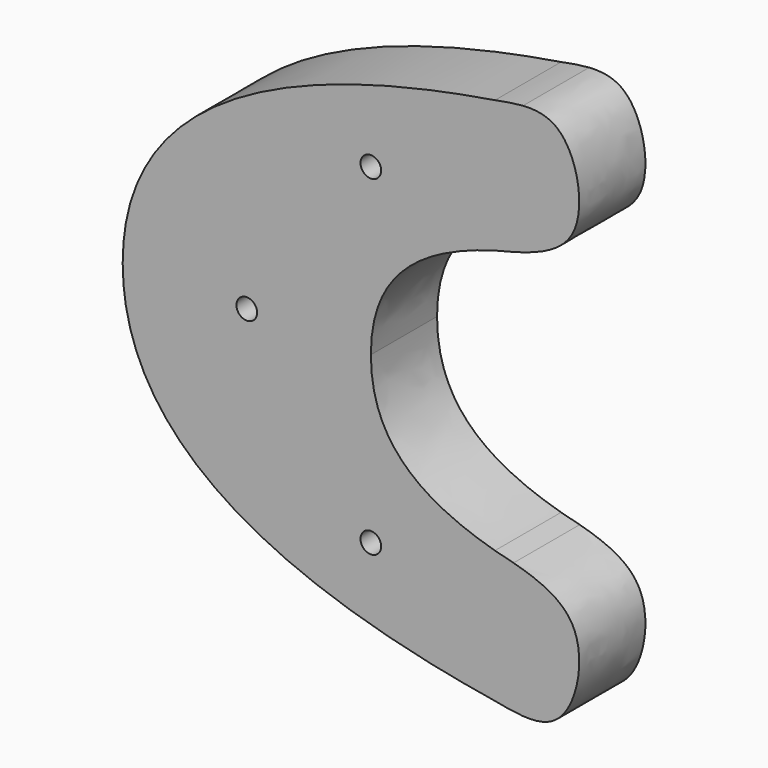
from build123d import *

# Parameters (mm, degrees)
F0_R     = 3.175
F1_DEPTH = 25.4


# Not quite as in the source:
# - ends of sketch curves that miss each other by under 0.0002 mm in the source are joined


with BuildPart() as f1:
    # F0 (on Front) → F1 (new body)
    with BuildSketch(Plane.XZ):
        with BuildLine():
            add(Edge.make_bspline(
                [(-228.6, 0), (-228.603328408, -20.9998549914), (-216.1362353399, -33.3187275092), (-190.5048638582, -40.5451878905)],
                knots=[0, 0, 0, 0, 96.8546122477, 96.8546122477, 96.8546122477, 96.8546122477], degree=3))
            add(Edge.make_bspline(
                [(-228.6, 0), (-228.603328408, 20.9998549914), (-216.1362353399, 33.3187275092), (-190.5048638582, 40.5451878905)],
                knots=[0, 0, 0, 0, 96.8546122477, 96.8546122477, 96.8546122477, 96.8546122477], degree=3))
            add(Edge.make_bspline(
                [(-190.5048638582, 40.5451878905), (-188.6690340196, 41.0627782819), (-186.7656708429, 41.5542443707), (-184.7945193799, 42.0209047272)],
                knots=[96.8546122477, 96.8546122477, 96.8546122477, 96.8546122477, 103.7917590678, 103.7917590678, 103.7917590678, 103.7917590678], degree=3))
            add(Edge.make_bspline(
                [(-181.8914412177, 82.4957251162), (-177.7740978469, 82.7671917451), (-166.6388871368, 81.1057466034), (-160.4841015231, 50.6684396177), (-176.6492852244, 44.2605429862), (-184.7945193799, 42.0209047272)],
                knots=[0.1201664208, 0.1201664208, 0.1201664208, 0.1201664208, 0.2987042421, 0.6454715168, 0.9336630859, 0.9336630859, 0.9336630859, 0.9336630859], degree=3))
            add(Edge.make_bspline(
                [(-190.5065755272, 81.190021553), (-187.6562706797, 81.6501805926), (-184.7832793111, 82.0849710788), (-181.8914412177, 82.4957251162)],
                knots=[152.2718692701, 152.2718692701, 152.2718692701, 152.2718692701, 159.2026765547, 159.2026765547, 159.2026765547, 159.2026765547], degree=3))
            add(Edge.make_bspline(
                [(-304.7999998765, 0.0020627141), (-304.7970834826, 48.7263819663), (-253.1268418931, 71.0804777771), (-190.5065755272, 81.190021553)],
                knots=[0.0042973705, 0.0042973705, 0.0042973705, 0.0042973705, 152.2718692701, 152.2718692701, 152.2718692701, 152.2718692701], degree=3))
            add(Edge.make_bspline(
                [(-304.8, -0.0020627142), (-304.8, -0.0006875504), (-304.7999999588, 0.0006875924), (-304.7999998765, 0.0020627141)],
                knots=[0, 0, 0, 0, 0.0042973705, 0.0042973705, 0.0042973705, 0.0042973705], degree=3))
            add(Edge.make_bspline(
                [(-304.8, -0.0020627142), (-304.7970834826, -48.7263819663), (-253.1268418931, -71.0804777771), (-190.5065755272, -81.190021553)],
                knots=[0.0042973705, 0.0042973705, 0.0042973705, 0.0042973705, 152.2718692701, 152.2718692701, 152.2718692701, 152.2718692701], degree=3))
            add(Edge.make_bspline(
                [(-190.5065755272, -81.190021553), (-187.6562706797, -81.6501805926), (-184.7832793111, -82.0849710788), (-181.8914412177, -82.4957251162)],
                knots=[152.2718692701, 152.2718692701, 152.2718692701, 152.2718692701, 159.2026765547, 159.2026765547, 159.2026765547, 159.2026765547], degree=3))
            add(Edge.make_bspline(
                [(-181.8914412177, -82.4957251162), (-177.7740978469, -82.7671917451), (-166.6388871368, -81.1057466034), (-160.4841015231, -50.6684396177), (-176.6492852244, -44.2605429862), (-184.7945193799, -42.0209047272)],
                knots=[0.1201664208, 0.1201664208, 0.1201664208, 0.1201664208, 0.2987042421, 0.6454715168, 0.9336630859, 0.9336630859, 0.9336630859, 0.9336630859], degree=3))
            add(Edge.make_bspline(
                [(-190.5048638582, -40.5451878905), (-188.6690340196, -41.0627782819), (-186.7656708429, -41.5542443707), (-184.7945193799, -42.0209047272)],
                knots=[96.8546122477, 96.8546122477, 96.8546122477, 96.8546122477, 103.7917590678, 103.7917590678, 103.7917590678, 103.7917590678], degree=3))
        make_face()
        with Locations((-228.6080516329, -50.8)):
            Circle(F0_R, mode=Mode.SUBTRACT)
        with Locations((-266.7, 0)):
            Circle(F0_R, mode=Mode.SUBTRACT)
        with Locations((-228.6080516329, 50.8)):
            Circle(F0_R, mode=Mode.SUBTRACT)
        with BuildLine():
            add(Edge.make_bspline(
                [(-190.5048638582, 40.5451878905), (-188.6690340196, 41.0627782819), (-186.7656708429, 41.5542443707), (-184.7945193799, 42.0209047272)],
                knots=[96.8546122477, 96.8546122477, 96.8546122477, 96.8546122477, 103.7917590678, 103.7917590678, 103.7917590678, 103.7917590678], degree=3))
            add(Edge.make_bspline(
                [(-184.7945193799, 42.0209047272), (-186.6694170397, 41.5053771867), (-188.587140449, 41.0252825386), (-190.5048638582, 40.5451878905)],
                knots=[0.9336630859, 0.9336630859, 0.9336630859, 0.9336630859, 1, 1, 1, 1], degree=3))
        make_face()
        with BuildLine():
            add(Edge.make_bspline(
                [(-184.7945193799, -42.0209047272), (-186.6694170397, -41.5053771867), (-188.587140449, -41.0252825386), (-190.5048638582, -40.5451878905)],
                knots=[0.9336630859, 0.9336630859, 0.9336630859, 0.9336630859, 1, 1, 1, 1], degree=3))
            add(Edge.make_bspline(
                [(-190.5048638582, -40.5451878905), (-188.6690340196, -41.0627782819), (-186.7656708429, -41.5542443707), (-184.7945193799, -42.0209047272)],
                knots=[96.8546122477, 96.8546122477, 96.8546122477, 96.8546122477, 103.7917590678, 103.7917590678, 103.7917590678, 103.7917590678], degree=3))
        make_face()
        with BuildLine():
            add(Edge.make_bspline(
                [(-190.5065755272, 81.190021553), (-187.6562706797, 81.6501805926), (-184.7832793111, 82.0849710788), (-181.8914412177, 82.4957251162)],
                knots=[152.2718692701, 152.2718692701, 152.2718692701, 152.2718692701, 159.2026765547, 159.2026765547, 159.2026765547, 159.2026765547], degree=3))
            add(Edge.make_bspline(
                [(-190.5065755272, 81.190021553), (-187.58461511, 81.7515168563), (-184.6626546928, 82.3130121597), (-181.8914412177, 82.4957251162)],
                knots=[0, 0, 0, 0, 0.1201664208, 0.1201664208, 0.1201664208, 0.1201664208], degree=3))
        make_face()
        with BuildLine():
            add(Edge.make_bspline(
                [(-190.5065755272, -81.190021553), (-187.58461511, -81.7515168563), (-184.6626546928, -82.3130121597), (-181.8914412177, -82.4957251162)],
                knots=[0, 0, 0, 0, 0.1201664208, 0.1201664208, 0.1201664208, 0.1201664208], degree=3))
            add(Edge.make_bspline(
                [(-190.5065755272, -81.190021553), (-187.6562706797, -81.6501805926), (-184.7832793111, -82.0849710788), (-181.8914412177, -82.4957251162)],
                knots=[152.2718692701, 152.2718692701, 152.2718692701, 152.2718692701, 159.2026765547, 159.2026765547, 159.2026765547, 159.2026765547], degree=3))
        make_face()
    extrude(amount=F1_DEPTH)


solid = f1.part
